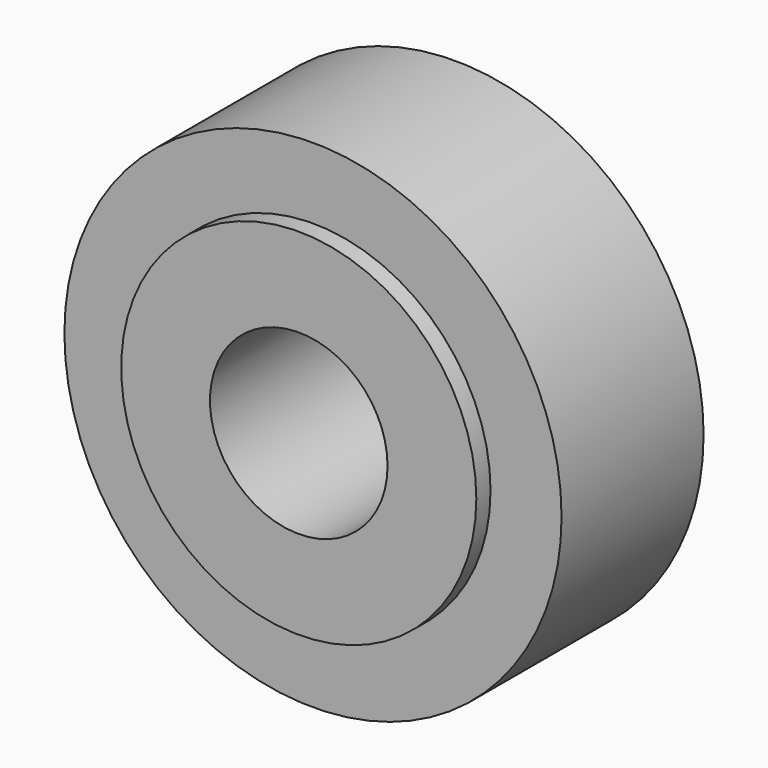
from build123d import *

# Parameters (mm, degrees)
F0_R     = 7
F0_R_2   = 2.5
F1_DEPTH = 5
F2_R     = 5
F2_R_2   = 2.5
F3_DEPTH = 0.5
F4_R     = 5
F4_R_2   = 2.5
F5_DEPTH = 0.5


with BuildPart() as f1:
    # F0 (on Front) → F1 (new body)
    with BuildSketch(Plane.XZ):
        Circle(F0_R)
        Circle(F0_R_2, mode=Mode.SUBTRACT)
    extrude(amount=F1_DEPTH)

    # F2 (on face) → F3 (join)
    with BuildSketch(Plane.XZ.offset(5)):
        Circle(F2_R)
        Circle(F2_R_2, mode=Mode.SUBTRACT)
    extrude(amount=F3_DEPTH)

    # F4 (on face) → F5 (join)
    with BuildSketch(Plane(origin=(0, 0, 0), x_dir=(-1, 0, 0), z_dir=(0, 1, 0))):
        Circle(F4_R)
        Circle(F4_R_2, mode=Mode.SUBTRACT)
    extrude(amount=F5_DEPTH)


solid = f1.part
